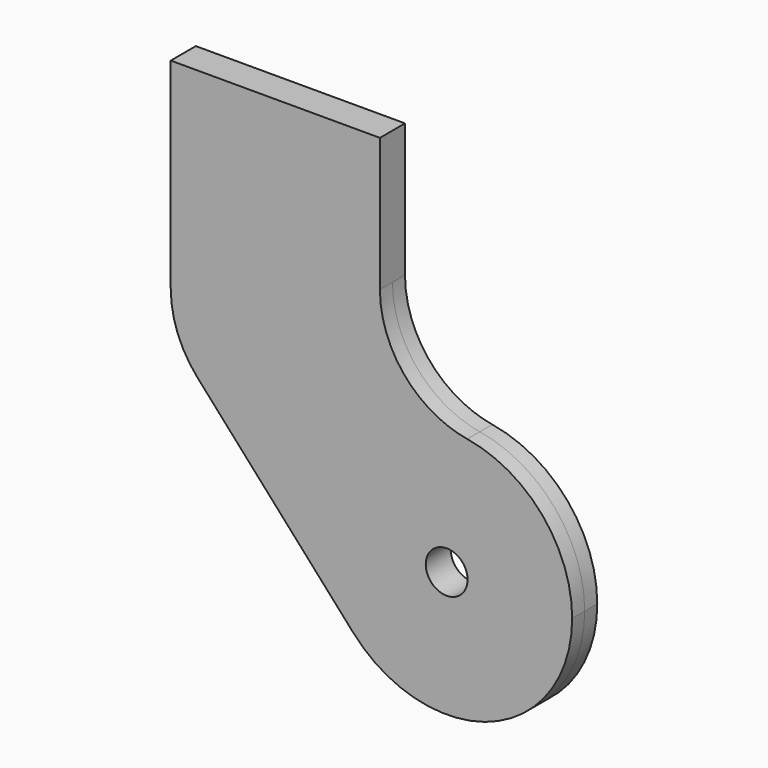
from build123d import *

# Parameters (mm, degrees)
F1_DEPTH = 4.7625
F3_D     = 12.7
F4_R     = 31.75


# Not quite as in the source:
# - a length typed as a fraction of an inch, garbled in the dataset ("3 / 203.2 mm" for 3/8 in), is restored


with BuildPart() as f1:
    # F0 (on Front) → F1 (new body, symmetric)
    with BuildSketch(Plane.XZ):
        with BuildLine():
            Line((31.75, -36.5125), (31.75, 36.5125))
            Line((31.75, 36.5125), (-31.75, 36.5125))
            Line((-31.75, 36.5125), (-31.75, -36.5125))
            Line((-31.75, -36.5125), (13.9433553622, -74.3740279097))
            ThreePointArc((13.9433553622, -74.3740279097), (19.5317526148, -53.0254697777), (36.0181289039, -38.3560964092))
            Line((36.0181289039, -38.3560964092), (31.75, -36.5125))
        make_face()
        with BuildLine():
            Line((62.0881194933, -49.616895256), (36.0181289039, -38.3560964092))
            ThreePointArc((36.0181289039, -38.3560964092), (19.5317526148, -53.0254697777), (13.9433553622, -74.3740279097))
            Line((13.9433553622, -74.3740279097), (35.8101662485, -92.4928739454))
            ThreePointArc((35.8101662485, -92.4928739454), (73.672422944, -86.207359662), (62.0881194933, -49.616895256))
        make_face()
        with BuildLine():
            ThreePointArc((48.5832224491, -34.9895780081), (42.1559369458, -36.1326186582), (36.0181289039, -38.3560964092))
            Line((36.0181289039, -38.3560964092), (62.0881194933, -49.616895256))
            ThreePointArc((62.0881194933, -49.616895256), (73.672422944, -86.207359662), (35.8101662485, -92.4928739454))
            Line((35.8101662485, -92.4928739454), (13.9433553622, -74.3740279097))
            ThreePointArc((13.9433553622, -74.3740279097), (16.6920555351, -87.2110882282), (23.6346841746, -98.3531426993))
            ThreePointArc((23.6346841746, -98.3531426993), (65.6226967812, -108.5221298326), (90.1161548124, -72.9346037083))
            ThreePointArc((90.1161548124, -72.9346037083), (77.7145523982, -44.8062841439), (48.5832224491, -34.9895780081))
        make_face()
        with BuildLine():
            Line((13.9433553622, -74.3740279097), (-31.75, -36.5125))
            Line((-31.75, -36.5125), (23.6346841746, -98.3531426993))
            ThreePointArc((23.6346841746, -98.3531426993), (16.6920555351, -87.2110882282), (13.9433553622, -74.3740279097))
        make_face()
        with BuildLine():
            Line((48.5832224491, -34.9895780081), (31.75, -36.5125))
            Line((31.75, -36.5125), (36.0181289039, -38.3560964092))
            ThreePointArc((36.0181289039, -38.3560964092), (42.1559369458, -36.1326186582), (48.5832224491, -34.9895780081))
        make_face()
    extrude(amount=F1_DEPTH, both=True)

    # F3 (through all)
    with Locations(Plane.XZ.offset(4.7625)):
        with Locations((52.0161548124, -72.9346037083)):
            Hole(F3_D / 2)

    # F4
    f4_edges = [f1.edges().sort_by_distance(p)[0] for p in [
        (-31.75, 0, -36.5125),
        (31.75, 0, -36.5125),
    ]]
    fillet(f4_edges, radius=F4_R)


solid = f1.part
